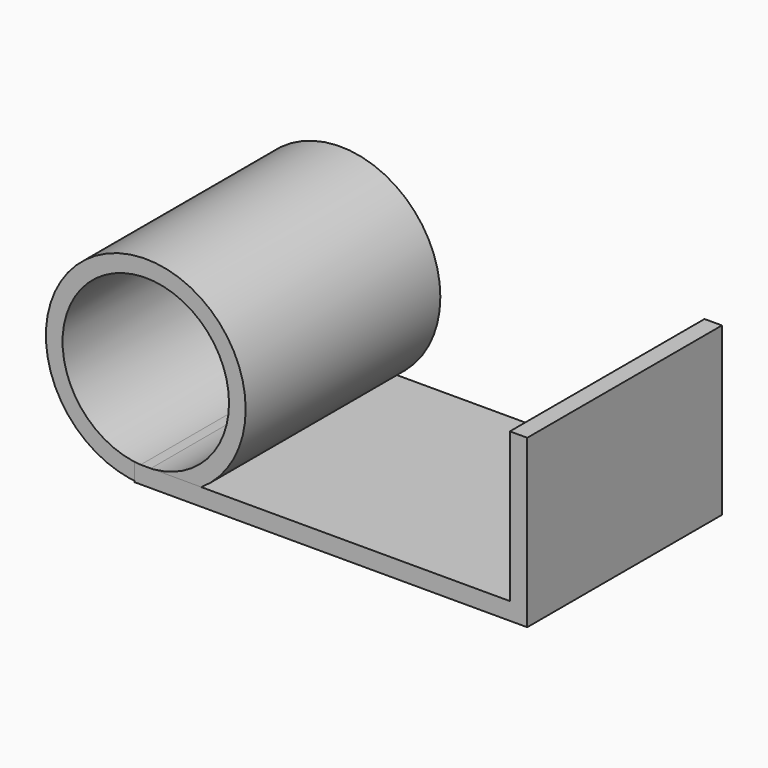
from build123d import *

# Parameters (mm, degrees)
F1_R     = 18.2467251248
F1_R_2   = 15.2039742304
F2_DEPTH = 44.45
F0_W     = 68.58
F0_H     = 3.175


with BuildPart() as f2:
    # F1 (on Front) → F2 (new body)
    with BuildSketch(Plane.XZ):
        with Locations((-41.5032282472, 15.1541987434)):
            Circle(F1_R)
        with Locations((-41.5032282472, 15.1541987434)):
            Circle(F1_R_2, mode=Mode.SUBTRACT)
    extrude(amount=F2_DEPTH)


with BuildPart() as f2b:
    # F0 (on Front) → F2, piece 2 (new body)
    with BuildSketch(Plane.XZ):
        with Locations((-9.2873283243, -1.5875)):
            Rectangle(F0_W, F0_H)
        Polygon((25.0026716757, 27.2931344807), (25.0026716757, 0), (25.0026716757, -3.175), (28.1776716757, -3.175), (28.1776716757, 27.2931344807), align=None)
    extrude(amount=F2_DEPTH)


solid = Compound([f2.part, f2b.part])
